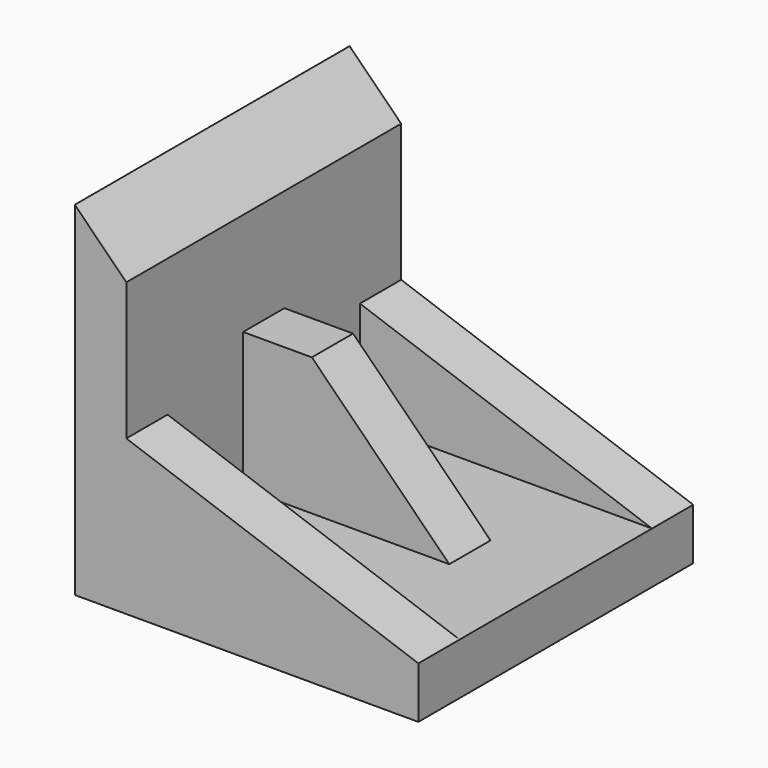
from build123d import *

# Parameters (mm, degrees)
F1_DEPTH = 127
F2_DEPTH = 19.05
F4_DEPTH = 38.1


# Not quite as in the source:
# - a pattern or mirror of a feature is missing from the dataset's text; its kind, count and spacing are read off the source's solid


with BuildPart() as f1:
    # F0 (on Front) → F1 (new body, symmetric)
    with BuildSketch(Plane.XZ):
        Polygon((0, 254), (0, 0), (254, 0), (254, 38.1), (190.5, 38.1), (38.1, 38.1), (38.1, 139.7), (38.1, 215.9), align=None)
    extrude(amount=F1_DEPTH, both=True)

    # F0 (on Front) → F2 (join, symmetric)
    with BuildSketch(Plane.XZ):
        Polygon((38.1, 38.1), (190.5, 38.1), (88.9, 139.7), (38.1, 139.7), align=None)
    extrude(amount=F2_DEPTH, both=True)

    # F3 (on face) → F4 (join)
    with BuildSketch(Plane.XZ.offset(127)):
        Polygon((254, 38.1), (38.1, 114.3), (38.1, 38.1), align=None)
    f4 = extrude(amount=-F4_DEPTH)

    # F4_copies: F4 across plane
    add(f4.mirror(Plane.ZX))


solid = f1.part
